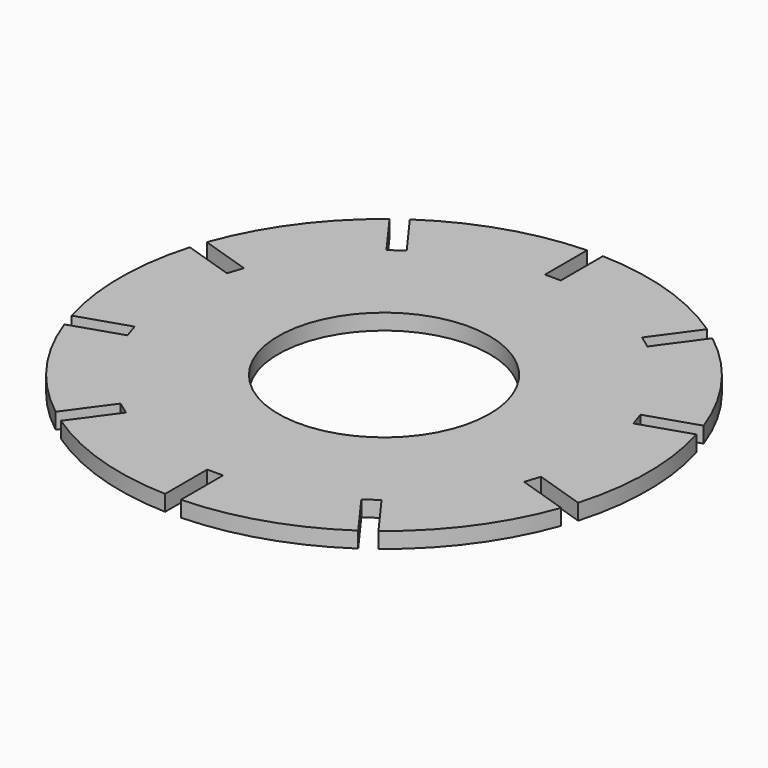
from build123d import *

# Parameters (mm, degrees)
F0_R            = 50
F0_R_2          = 20
F2_DEPTH        = 3
F1_W            = 3
F1_H            = 10
F3_DEPTH        = 25
F3_COPIES_COUNT = 10


# Not quite as in the source:
# - a pattern or mirror of a feature is missing from the dataset's text; its kind, count and spacing are read off the source's solid


with BuildPart() as f2:
    # F0 (on Top) → F2 (new body)
    with BuildSketch(Plane.XY):
        Circle(F0_R)
        Circle(F0_R_2, mode=Mode.SUBTRACT)
    extrude(amount=F2_DEPTH)

    # F1 (on Top) → F3 (cut)
    with BuildSketch(Plane.XY):
        with Locations((0, 45)):
            Rectangle(F1_W, F1_H)
    f3 = extrude(amount=F3_DEPTH, mode=Mode.SUBTRACT)

    # F3_copies: F3 ×10 about axis
    f3_copies_axis = Axis((0, 0, 0), (0, 0, 1))
    for i in range(1, F3_COPIES_COUNT):
        add(f3.rotate(f3_copies_axis, i * 360 / F3_COPIES_COUNT), mode=Mode.SUBTRACT)


solid = f2.part
